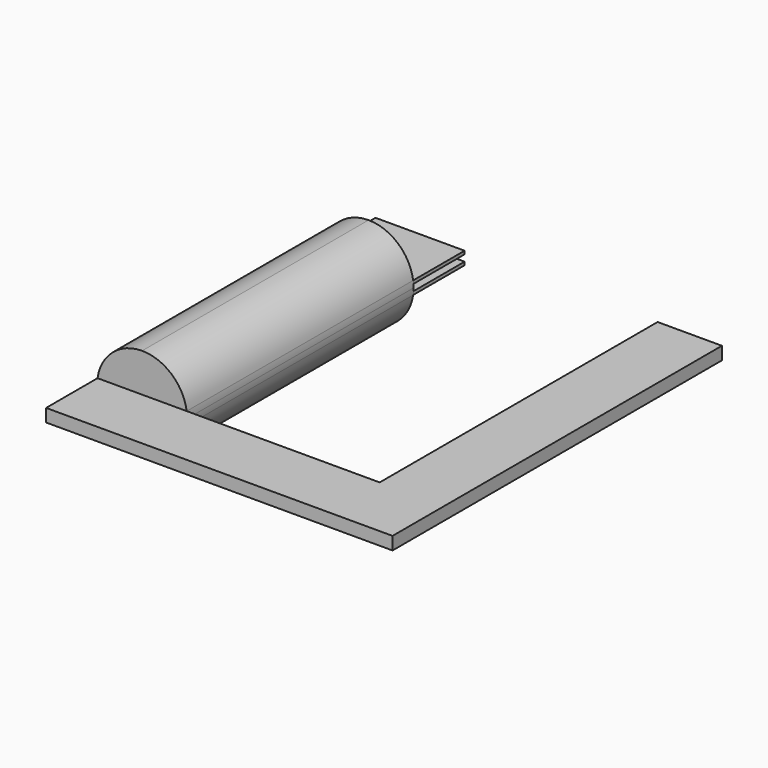
from build123d import *

# Parameters (mm, degrees)
F1_DEPTH  = 22
F3_DEPTH  = 5
F5_DEPTH  = 5
F7_DEPTH  = 25
F8_DEPTH  = 20
F9_W      = 5
F9_H      = 1
F10_DEPTH = 27
F11_W     = 5
F11_H     = 0.5
F12_DEPTH = 1
F13_W     = 5
F13_H     = 0.5
F14_DEPTH = 1


with BuildPart() as f1:
    # F0 (on Front) → F1 (new body)
    with BuildSketch(Plane.XZ):
        with BuildLine():
            ThreePointArc((0, -3.5), (2.4748737342, -2.4748737342), (3.5, 0))
            ThreePointArc((3.5, 0), (2.4748737342, 2.4748737342), (0, 3.5))
            ThreePointArc((0, 3.5), (-2.4748737342, 2.4748737342), (-3.5, 0))
            ThreePointArc((-3.5, 0), (-2.4748737342, -2.4748737342), (0, -3.5))
        make_face()
        with BuildLine():
            ThreePointArc((-3.5, 0), (-2.4748737342, 2.4748737342), (0, 3.5))
            Line((0, 3.5), (-3.5, 3.5))
            Line((-3.5, 3.5), (-3.5, 0))
        make_face()
        with BuildLine():
            Line((-3.5, -3.5), (0, -3.5))
            ThreePointArc((0, -3.5), (-2.4748737342, -2.4748737342), (-3.5, 0))
            Line((-3.5, 0), (-3.5, -3.5))
        make_face()
        with BuildLine():
            Line((3.5, -3.5), (3.5, 0))
            ThreePointArc((3.5, 0), (2.4748737342, -2.4748737342), (0, -3.5))
            Line((0, -3.5), (3.5, -3.5))
        make_face()
        with BuildLine():
            ThreePointArc((0, 3.5), (2.4748737342, 2.4748737342), (3.5, 0))
            Line((3.5, 0), (3.5, 3.5))
            Line((3.5, 3.5), (0, 3.5))
        make_face()
    extrude(amount=F1_DEPTH)

    # F2 (on face) → F3 (join)
    with BuildSketch(Plane.XZ.offset(22)):
        Polygon((3.4641016151, -0.5), (3.4641016151, 0.5), (0, 0.5), (-3.4641016151, 0.5), (-3.4641016151, -0.5), align=None)
    extrude(amount=F3_DEPTH)

    # F4 (on face) → F5 (join)
    with BuildSketch(Plane(origin=(0, 0, 0), x_dir=(-1, 0, 0), z_dir=(0, 1, 0))):
        Polygon((3.4641016151, -0.5), (3.4641016151, 0.5), (0, 0.5), (-3.4641016151, 0.5), (-3.4641016151, -0.5), (0, -0.5), align=None)
    extrude(amount=F5_DEPTH)

    # F6 (on face) → F7 (cut)
    with BuildSketch(Plane(origin=(0, 0, 0), x_dir=(-1, 0, 0), z_dir=(0, 1, 0))):
        with BuildLine():
            ThreePointArc((-3.4641016151, 0.5), (-2.2912878475, 2.6457513111), (0, 3.5))
            Line((0, 3.5), (-3.5, 3.5))
            Line((-3.5, 3.5), (-3.5, 0))
            ThreePointArc((-3.5, 0), (-3.491013868, 0.2506435188), (-3.4641016151, 0.5))
        make_face()
        with BuildLine():
            ThreePointArc((3.4641016151, 0.5), (3.491013868, 0.2506435188), (3.5, 0))
            Line((3.5, 0), (3.5, 3.5))
            Line((3.5, 3.5), (0, 3.5))
            ThreePointArc((0, 3.5), (2.2912878475, 2.6457513111), (3.4641016151, 0.5))
        make_face()
        with BuildLine():
            Line((-3.5, -3.5), (0, -3.5))
            ThreePointArc((0, -3.5), (-2.2912878475, -2.6457513111), (-3.4641016151, -0.5))
            ThreePointArc((-3.4641016151, -0.5), (-3.491013868, -0.2506435188), (-3.5, 0))
            Line((-3.5, 0), (-3.5, -3.5))
        make_face()
        with BuildLine():
            Line((3.5, -3.5), (3.5, 0))
            ThreePointArc((3.5, 0), (3.491013868, -0.2506435188), (3.4641016151, -0.5))
            ThreePointArc((3.4641016151, -0.5), (2.2912878475, -2.6457513111), (0, -3.5))
            Line((0, -3.5), (3.5, -3.5))
        make_face()
    extrude(amount=-F7_DEPTH, mode=Mode.SUBTRACT)

    # F8 (add): a face of the model
    f8_faces = [f1.faces().sort_by_distance(p)[0] for p in [
        (3.4641016151, -24.5, 0),
    ]]
    extrude(f8_faces, amount=F8_DEPTH)

    # F9 (on face) → F10 (join)
    with BuildSketch(Plane(origin=(0, -22, 0), x_dir=(-1, 0, 0), z_dir=(0, 1, 0))):
        with Locations((-20.9641016151, 0)):
            Rectangle(F9_W, F9_H)
    extrude(amount=F10_DEPTH)

    # F11 (on face) → F12 (cut)
    with BuildSketch(Plane(origin=(18.4641016151, 0, 0), x_dir=(0, -1, 0), z_dir=(-1, 0, 0))):
        with Locations((-2.5, 0)):
            Rectangle(F11_W, F11_H)
    extrude(amount=-F12_DEPTH, mode=Mode.SUBTRACT)

    # F13 (on face) → F14 (cut)
    with BuildSketch(Plane.YZ.offset(3.4641016151)):
        with Locations((2.5, 0)):
            Rectangle(F13_W, F13_H)
    extrude(amount=-F14_DEPTH, mode=Mode.SUBTRACT)


solid = f1.part
